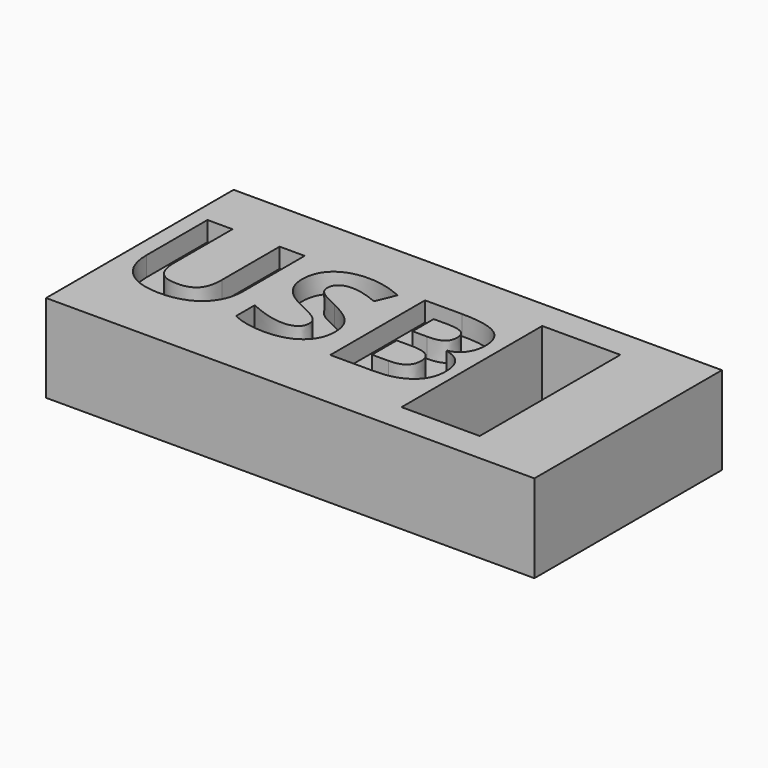
from build123d import *

# Parameters (mm, degrees)
F0_W         = 25
F0_H         = 12
F1_DEPTH     = 4.5
F2_W         = 4
F2_H         = 9
F3_DEPTH     = 25
F4_TEXT_SIZE = 8.4912876547
F5_DEPTH     = 1


# Not quite as in the source:
# - Text() gives the source's letters only with a copy of the font that has no kerning and outlines rounded to 1/6400 em; it was checked with that copy


with BuildPart() as f1:
    # F0 (on Top) → F1 (new body)
    with BuildSketch(Plane.XY):
        Rectangle(F0_W, F0_H)
    extrude(amount=F1_DEPTH)

    # F2 (on face) → F3 (cut)
    with BuildSketch(Plane.XY.offset(4.5)):
        with Locations((6.5, 0)):
            Rectangle(F2_W, F2_H)
    extrude(amount=-F3_DEPTH, mode=Mode.SUBTRACT)

    # F4 (on face) → F5 (cut)
    with BuildSketch(Plane.XY.offset(4.5)):
        with Locations((-12.4042962513, -2.7554933913)):
            Text('USB', F4_TEXT_SIZE, font='Open Sans', font_style=FontStyle.BOLD, text_align=(TextAlign.LEFT, TextAlign.BOTTOM))
    extrude(amount=-F5_DEPTH, mode=Mode.SUBTRACT)


solid = f1.part
